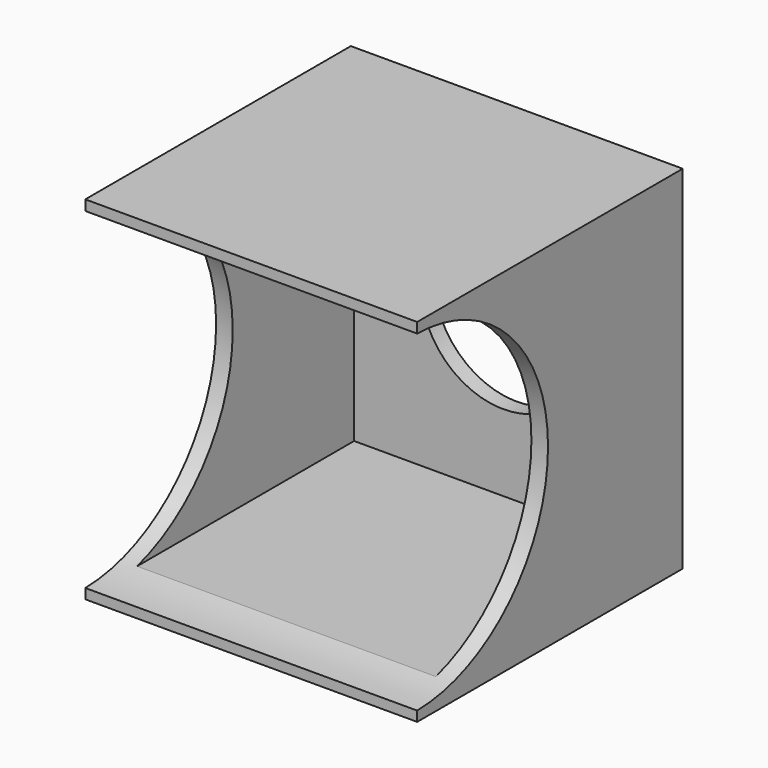
from build123d import *

# Parameters (mm, degrees)
F0_W     = 50
F0_H     = 53.0426052851
F1_DEPTH = 50
F2_R     = 25
F3_DEPTH = 25
F4_DEPTH = 25
F5_T     = 2.5
F6_R     = 12.5
F7_DEPTH = 50


# Not quite as in the source:
# - a shell that OpenCascade refuses in one call is made with other operations: the cavity is built on its own and cut out


with BuildPart() as f1:
    # F0 (on Front) → F1 (new body)
    with BuildSketch(Plane.XZ):
        Rectangle(F0_W, F0_H)
    extrude(amount=-F1_DEPTH)

    # F2 (on Right) → F3 (cut)
    with BuildSketch(Plane.YZ):
        with Locations((-0.3665760159, -0.021956861)):
            Circle(F2_R)
    extrude(amount=F3_DEPTH, mode=Mode.SUBTRACT)

    # F2 (on Right) → F4 (cut)
    with BuildSketch(Plane.YZ):
        with Locations((-0.3665760159, -0.021956861)):
            Circle(F2_R)
    extrude(amount=-F4_DEPTH, mode=Mode.SUBTRACT)

    # F5: shell of thickness 2.5, made by hand


with BuildPart() as f5_core1:
    # F5_t2: copy of F1
    add(f1.part)

    # the walls: a layer under each face that stays
    f5_faces = [f5_core1.faces().sort_by_distance(p)[0] for p in [
        (-25, 25, 0),
        (25, 25, 0),
        (0, 0, -25.7702858998),
        (0, 25, -26.5213026426),
        (0, 50, 0),
        (0, 25, 26.5213026426),
        (0, 0, 25.7483290388),
    ]]
    thicken(f5_faces, amount=-F5_T, mode=Mode.SUBTRACT)


with BuildPart() as f1_1:
    add(f1.part)

    # what is left inside the walls is the cavity
    f5_cavity = [f5_core1.part.solids().sort_by_distance(p)[0] for p in [
        (-7.5, 24.658298, 0.057376),
    ]]
    add(f5_cavity, mode=Mode.SUBTRACT)

    # F6 (on Front) → F7 (cut)
    with BuildSketch(Plane.XZ):
        Circle(F6_R)
    extrude(amount=-F7_DEPTH, mode=Mode.SUBTRACT)


solid = f1_1.part
